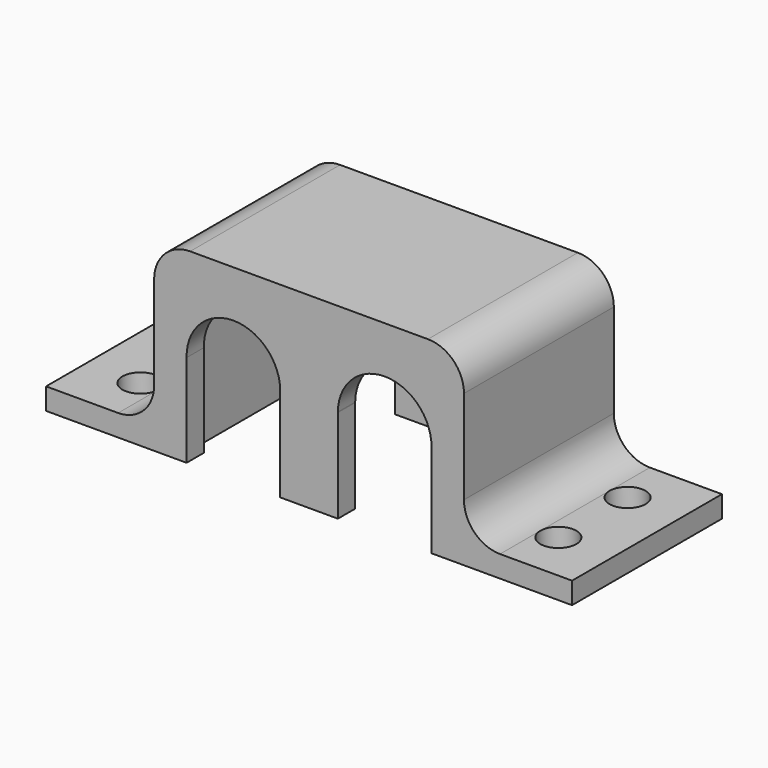
from build123d import *

# Parameters (mm, degrees)
F1_W          = 43
F1_H          = 26
F2_DEPTH      = 13
F2_DEPTH_BACK = 13
F3_T          = -3
F5_W          = 15
F5_H          = 26
F5_R          = 2.5
F5_W_2        = 43
F5_W_3        = 37
F5_H_2        = 20
F6_DEPTH      = 3
F7_R          = 4.99999
F9_DEPTH      = 5
F10_DEPTH     = 25


# Not quite as in the source:
# - a fillet or chamfer is up to 0.001 mm smaller than in the source, because OpenCascade refuses the exact size


with BuildPart() as f2:
    # F1 (on Top) → F2 (new body, two sides)
    with BuildSketch(Plane.XY) as f2_sk:
        with Locations((0, 13)):
            Rectangle(F1_W, F1_H)
    extrude(amount=F2_DEPTH)
    extrude(f2_sk.sketch, amount=-F2_DEPTH_BACK)

    # F3
    f3_openings = [f2.faces().sort_by_distance(p)[0] for p in [
        (0, 13, -13),
    ]]
    offset(amount=F3_T, openings=f3_openings)

    # F5 (on face) → F6 (join)
    with BuildSketch(Plane(origin=(0, 0, -13), x_dir=(1, 0, 0), z_dir=(0, 0, -1))):
        with Locations((-29, -13)):
            Rectangle(F5_W, F5_H)
        with Locations((-29, -19)):
            Circle(F5_R, mode=Mode.SUBTRACT)
        with Locations((-29, -7)):
            Circle(F5_R, mode=Mode.SUBTRACT)
        with Locations((0, -13)):
            Rectangle(F5_W_2, F5_H)
        with Locations((0, -13)):
            Rectangle(F5_W_3, F5_H_2, mode=Mode.SUBTRACT)
        with Locations((29, -13)):
            Rectangle(F5_W, F5_H)
        with Locations((29, -19)):
            Circle(F5_R, mode=Mode.SUBTRACT)
        with Locations((29, -7)):
            Circle(F5_R, mode=Mode.SUBTRACT)
    extrude(amount=-F6_DEPTH)

    # F7 (radius 5 in the source; OpenCascade refuses exactly that, so slightly less here)
    f7_edges = [f2.edges().sort_by_distance(p)[0] for p in [
        (-21.5, 13, 13),
        (21.5, 13, 13),
        (-21.5, 13, -10),
        (21.5, 13, -10),
        (0, 23, 10),
        (0, 3, 10),
        (-18.5, 13, 10),
        (18.5, 13, 10),
    ]]
    fillet(f7_edges, radius=F7_R)

    # F8 (on face) → F9 (cut)
    with BuildSketch(Plane.XZ):
        with BuildLine():
            Line((-4.0000936475, -11), (-4.0000936475, -0.0348913798))
            ThreePointArc((-4.0000936475, -0.0348913798), (-4, 0), (-4.0000936475, 0.0348913798))
            ThreePointArc((-4.0000936475, 0.0348913798), (-10.5909716955, 6.499363365), (-16.9983365331, -0.1470452389))
            Line((-16.9983365331, -0.1470452389), (-16.9983365331, -10.9773843356))
            Line((-16.9983365331, -10.9773843356), (-16.9983365331, -13))
            Line((-16.9983365331, -13), (-4.0000936475, -13))
            Line((-4.0000936475, -13), (-4.0000936475, -11))
        make_face()
        with BuildLine():
            ThreePointArc((4.0000936475, 0.0348913798), (4, 0), (4.0000936475, -0.0348913798))
            Line((4.0000936475, -0.0348913798), (4.0000936475, -11))
            Line((4.0000936475, -11), (4.0000936475, -13))
            Line((4.0000936475, -13), (16.9983365331, -13))
            Line((16.9983365331, -13), (16.9983365331, -10.9773843356))
            Line((16.9983365331, -10.9773843356), (16.9983365331, -0.1470452389))
            ThreePointArc((16.9983365331, -0.1470452389), (10.5909716955, 6.499363365), (4.0000936475, 0.0348913798))
        make_face()
    extrude(amount=-F9_DEPTH, mode=Mode.SUBTRACT)

    # F4 (on face) → F10 (cut)
    with BuildSketch(Plane(origin=(0, 26, 0), x_dir=(-1, 0, 0), z_dir=(0, 1, 0))):
        with BuildLine():
            Line((-6.5, -13), (-6.5, 0))
            ThreePointArc((-6.5, 0), (-10.5, 4), (-14.5, 0))
            Line((-14.5, 0), (-14.5, -13))
            Line((-14.5, -13), (-6.5, -13))
        make_face()
        with BuildLine():
            ThreePointArc((14.5, 0), (10.5, 4), (6.5, 0))
            Line((6.5, 0), (6.5, -13))
            Line((6.5, -13), (14.5, -13))
            Line((14.5, -13), (14.5, 0))
        make_face()
    extrude(amount=-F10_DEPTH, mode=Mode.SUBTRACT)


solid = f2.part
